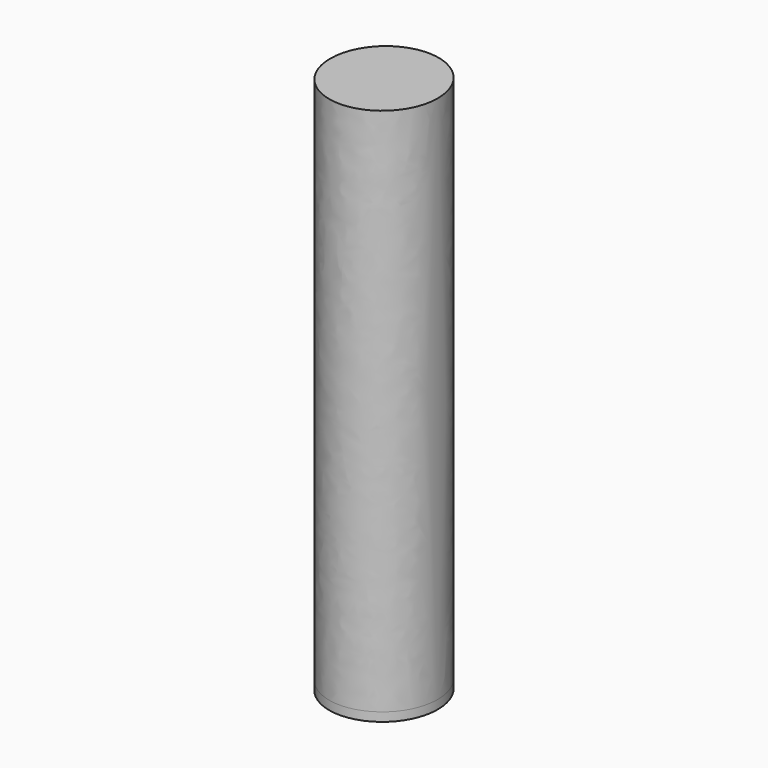
from build123d import *

# Parameters (mm, degrees)
F1_DEPTH      = 762
F1_DEPTH_BACK = 12.7
F2_R          = 61.0536271801
F3_DEPTH      = 736.6


# Not quite as in the source:
# - a length typed as a fraction of an inch, garbled in the dataset ("3 / 203.2 mm" for 3/8 in), is restored


with BuildPart() as f1:
    # F0 (on Top) → F1 (new body, two sides)
    with BuildSketch(Plane.XY) as f1_sk:
        with BuildLine():
            add(Edge.make_bspline(
                [(77.4405226111, 0), (77.4405226111, 137.9003787083), (-38.7202613056, 68.9501893541), (-154.8810452223, 0), (-38.7202613056, -68.9501893541), (77.4405226111, -137.9003787083), (77.4405226111, 0)],
                knots=[4.7123889804, 4.7123889804, 4.7123889804, 6.8067840828, 6.8067840828, 8.9011791852, 8.9011791852, 10.9955742876, 10.9955742876, 10.9955742876], degree=2, weights=[1, 0.5, 1, 0.5, 1, 0.5, 1]))
        make_face()
    extrude(amount=F1_DEPTH)
    extrude(f1_sk.sketch, amount=-F1_DEPTH_BACK)

    # F2 (on face) → F3 (join)
    with BuildSketch(Plane.XY.offset(762)):
        Circle(F2_R)
    extrude(amount=-F3_DEPTH)


solid = f1.part
